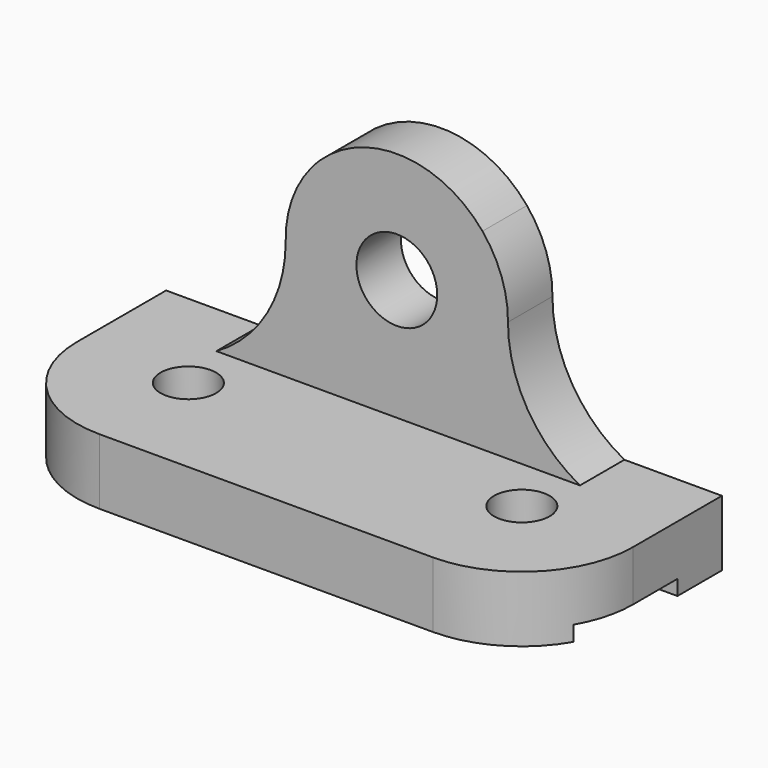
from build123d import *

# Parameters (mm, degrees)
F1_DEPTH  = 1117.6
F2_R      = 76.2
F3_W      = 838.2
F3_H      = 1016.8327547744
F4_DEPTH  = 889
F5_R      = 139.7
F6_DEPTH  = 330.2
F8_DEPTH  = 330.2
F10_DEPTH = 279.4
F12_DEPTH = 279.4
F13_R     = 203.2
F14_DEPTH = 279.4
F16_DEPTH = 279.4
F17_W     = 279.4
F17_H     = 76.2
F18_DEPTH = 2794


# Not quite as in the source:
# - after a boolean that leaves OpenCascade's solid faulty, fix() repairs it


with BuildPart() as f1:
    # F0 (on Front) → F1 (new body)
    with BuildSketch(Plane.XZ):
        with BuildLine():
            Line((-1656.6551755185, 330.2), (-1656.6551755185, 0))
            Line((-1656.6551755185, 0), (1137.3448244815, 0))
            Line((1137.3448244815, 0), (1137.3448244815, 330.2))
            Line((1137.3448244815, 330.2), (157.1546553156, 330.2))
            Line((157.1546553156, 330.2), (157.1546553156, 1347.0327547744))
            Line((157.1546553156, 1347.0327547744), (-697.5968859522, 1347.0327547744))
            ThreePointArc((-697.5968859522, 1347.0327547744), (-702.0870140127, 1345.1728828349), (-703.9468859522, 1340.6827547744))
            Line((-703.9468859522, 1340.6827547744), (-703.9468859522, 330.2))
            Line((-703.9468859522, 330.2), (-1656.6551755185, 330.2))
        make_face()
    extrude(amount=F1_DEPTH)

    # F2
    f2_edges = [f1.edges().sort_by_distance(p)[0] for p in [
        (-1656.655176, -1117.6, 165.1),
        (1137.344824, -1117.6, 165.1),
    ]]
    fillet(f2_edges, radius=F2_R)

    # F3 (on face) → F4 (cut)
    with BuildSketch(Plane.YZ.offset(157.1546553156)):
        with Locations((-698.5, 838.6163773872)):
            Rectangle(F3_W, F3_H)
    extrude(amount=-F4_DEPTH, mode=Mode.SUBTRACT)

    # F5 (on face) → F6 (cut)
    with BuildSketch(Plane.XY.offset(330.2)):
        with BuildLine():
            ThreePointArc((718.2448244815, -558.8), (578.5448244815, -419.1), (438.8448244815, -558.8))
            ThreePointArc((438.8448244815, -558.8), (578.5448244815, -698.5), (718.2448244815, -558.8))
        make_face()
        with Locations((-1097.8551755185, -558.8)):
            Circle(F5_R)
    extrude(amount=-F6_DEPTH, mode=Mode.SUBTRACT)

    # F7 (on face) → F8 (cut)
    with BuildSketch(Plane.XY.offset(330.2)):
        with BuildLine():
            Line((-1580.4551755185, -1117.6), (-1097.8551755185, -1117.6))
            ThreePointArc((-1097.8551755185, -1117.6), (-1492.9864448455, -953.931269327), (-1656.6551755185, -558.8))
            Line((-1656.6551755185, -558.8), (-1656.6551755185, -1041.4))
            ThreePointArc((-1656.6551755185, -1041.4), (-1634.3367122449, -1095.2815367264), (-1580.4551755185, -1117.6))
        make_face()
        with BuildLine():
            ThreePointArc((1137.3448244815, -558.8), (973.6760925431, -953.9312705925), (578.5448209022, -1117.6))
            Line((578.5448209022, -1117.6), (1061.1448244815, -1117.6))
            ThreePointArc((1061.1448244815, -1117.6), (1115.026361208, -1095.2815367264), (1137.3448244815, -1041.4))
            Line((1137.3448244815, -1041.4), (1137.3448244815, -558.8))
        make_face()
    extrude(amount=-F8_DEPTH, mode=Mode.SUBTRACT)

    # F9 (on face) → F10 (cut)
    with BuildSketch(Plane.XZ.offset(279.4)):
        with BuildLine():
            Line((-703.9468859522, 1340.6827547744), (-703.9468859522, 1296.0070660537))
            ThreePointArc((-703.9468859522, 1296.0070660537), (-680.7947693951, 1322.2706219521), (-656.0433725133, 1347.0327547744))
            Line((-656.0433725133, 1347.0327547744), (-697.5968859522, 1347.0327547744))
            ThreePointArc((-697.5968859522, 1347.0327547744), (-702.0870140127, 1345.1728828349), (-703.9468859522, 1340.6827547744))
        make_face()
        with BuildLine():
            ThreePointArc((109.2511418767, 1347.0327547744), (134.0025387585, 1322.2706219521), (157.1546553156, 1296.0070660537))
            Line((157.1546553156, 1296.0070660537), (157.1546553156, 1347.0327547744))
            Line((157.1546553156, 1347.0327547744), (109.2511418767, 1347.0327547744))
        make_face()
    extrude(amount=-F10_DEPTH, mode=Mode.SUBTRACT)

    # F11 (on face) → F12 (join)
    with BuildSketch(Plane.XZ.offset(279.4)):
        with BuildLine():
            Line((-703.9468859522, 330.2), (-273.3961153183, 330.2))
            Line((-273.3961153183, 330.2), (-273.3961153183, 381))
            ThreePointArc((-273.3961153183, 381), (-511.3130456629, 434.1786255948), (-703.9468859522, 583.5929339463))
            Line((-703.9468859522, 583.5929339463), (-703.9468859522, 330.2))
        make_face()
        with BuildLine():
            Line((-273.3961153183, 381), (-273.3961153183, 330.2))
            Line((-273.3961153183, 330.2), (157.1546553156, 330.2))
            Line((157.1546553156, 330.2), (157.1546553156, 583.5929339463))
            ThreePointArc((157.1546553156, 583.5929339463), (-35.4791849737, 434.1786255948), (-273.3961153183, 381))
        make_face()
        with BuildLine():
            ThreePointArc((-703.9468859522, 583.5929339463), (-511.3130456629, 434.1786255948), (-273.3961153183, 381))
            ThreePointArc((-273.3961153183, 381), (-35.4791849737, 434.1786255948), (157.1546553156, 583.5929339463))
            Line((157.1546553156, 583.5929339463), (157.1546553156, 1296.0070660537))
            ThreePointArc((157.1546553156, 1296.0070660537), (134.0025387585, 1322.2706219521), (109.2511418767, 1347.0327547744))
            Line((109.2511418767, 1347.0327547744), (-656.0433725133, 1347.0327547744))
            ThreePointArc((-656.0433725133, 1347.0327547744), (-680.7947693951, 1322.2706219521), (-703.9468859522, 1296.0070660537))
            Line((-703.9468859522, 1296.0070660537), (-703.9468859522, 583.5929339463))
        make_face()
        with BuildLine():
            ThreePointArc((-703.9468859522, 1296.0070660537), (-832.1961153183, 939.8), (-703.9468859522, 583.5929339463))
            Line((-703.9468859522, 583.5929339463), (-703.9468859522, 1296.0070660537))
        make_face()
        with BuildLine():
            Line((157.1546553156, 1296.0070660537), (157.1546553156, 583.5929339463))
            ThreePointArc((157.1546553156, 583.5929339463), (252.3648620422, 750.504372251), (285.4038846817, 939.8))
            ThreePointArc((285.4038846817, 939.8), (252.3648620422, 1129.095627749), (157.1546553156, 1296.0070660537))
        make_face()
        with BuildLine():
            ThreePointArc((109.2511418767, 1347.0327547744), (-273.3961153183, 1498.6), (-656.0433725133, 1347.0327547744))
            Line((-656.0433725133, 1347.0327547744), (109.2511418767, 1347.0327547744))
        make_face()
    extrude(amount=-F12_DEPTH)

    add(f1.part.fix(), mode=Mode.REPLACE)

    # F13 (on face) → F14 (cut)
    with BuildSketch(Plane.XZ.offset(279.4)):
        with Locations((-273.3961153183, 939.8)):
            Circle(F13_R)
    extrude(amount=-F14_DEPTH, mode=Mode.SUBTRACT)

    # F15 (on face) → F16 (join)
    with BuildSketch(Plane(origin=(0, 0, 0), x_dir=(-1, 0, 0), z_dir=(0, 1, 0))):
        with BuildLine():
            ThreePointArc((-285.3849203754, 935.1962896365), (-285.390539451, 937.4981607316), (-285.4038846817, 939.8))
            ThreePointArc((-285.4038846817, 939.8), (-285.399143585, 937.4981252882), (-285.3849203754, 935.1962896365))
        make_face()
        with BuildLine():
            ThreePointArc((-157.1546553156, 583.5929339463), (-251.5806324391, 748.3402018334), (-285.3849203754, 935.1962896365))
            ThreePointArc((-285.3849203754, 935.1962896365), (-382.6303819595, 582.6426933759), (-647.2497398986, 330.2))
            Line((-647.2497398986, 330.2), (-157.1546553156, 330.2))
            Line((-157.1546553156, 330.2), (-157.1546553156, 583.5929339463))
        make_face()
        with BuildLine():
            ThreePointArc((1180.3010307353, 330.2), (925.1728780454, 582.1676650218), (832.0808509298, 928.4507183164))
            ThreePointArc((832.0808509298, 928.4507183164), (797.2075743036, 745.174730737), (703.9468859522, 583.5929339463))
            Line((703.9468859522, 583.5929339463), (703.9468859522, 330.2))
            Line((703.9468859522, 330.2), (1180.3010307353, 330.2))
        make_face()
    extrude(amount=-F16_DEPTH)

    # F17 (on face) → F18 (cut)
    with BuildSketch(Plane.YZ.offset(1137.3448244815)):
        with Locations((-419.1, 38.1)):
            Rectangle(F17_W, F17_H)
        with Locations((-698.5, 38.1)):
            Rectangle(F17_W, F17_H)
    extrude(amount=-F18_DEPTH, mode=Mode.SUBTRACT)


solid = f1.part
